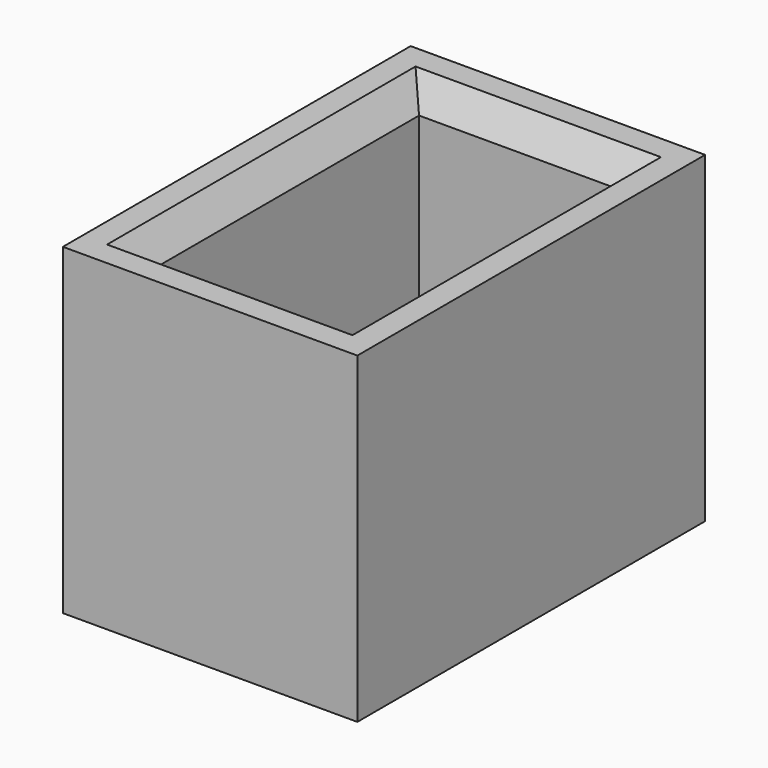
from build123d import *

# Parameters (mm, degrees)
F0_W         = 6
F0_H         = 10
F1_DEPTH     = 8
F2_T         = 1.2
F3_T1_DEPTH  = 6
F3_T3_DEPTH  = 10
F3_T9_DEPTH  = 8.2404819853
F3_T13_DEPTH = 12.2404819853
F3_T20_DEPTH = 8.2404819853
F3_T24_DEPTH = 12.2404819853
F3_T31_DEPTH = 12.2404819853
F3_T35_DEPTH = 8.2404819853
F3_T42_DEPTH = 8.2404819853
F3_T46_DEPTH = 12.2404819853


# Not quite as in the source:
# - a fillet or chamfer that OpenCascade refuses, or shapes differently, is made with other operations: its cross-section is extruded or revolved along the edge and cut away or added


with BuildPart() as f1:
    # F0 (on Top) → F1 (new body)
    with BuildSketch(Plane.XY):
        Rectangle(F0_W, F0_H)
    extrude(amount=F1_DEPTH)

    # F2
    f2_openings = [f1.faces().sort_by_distance(p)[0] for p in [
        (0, 0, 8),
    ]]
    offset(amount=F2_T, openings=f2_openings, kind=Kind.INTERSECTION)

    # F3: chamfer of 0.5 x 0.8660254038 on 4 edges, made by hand

    # F3_s2 → F3_t1 (cut)
    with BuildSketch(Plane.YZ.offset(-3)):
        Polygon((5, 7.1339745962), (5.5, 8), (5, 8), align=None)
        Polygon((-5, 7.1339745962), (-5.5, 8), (-5, 8), align=None)
    extrude(amount=F3_T1_DEPTH, mode=Mode.SUBTRACT)

    # F3_s4 → F3_t3 (cut)
    with BuildSketch(Plane.XZ.offset(-5)):
        Polygon((-3, 7.1339745962), (-3.5, 8), (-3, 8), align=None)
        Polygon((3, 7.1339745962), (3.5, 8), (3, 8), align=None)
    extrude(amount=F3_T3_DEPTH, mode=Mode.SUBTRACT)


with BuildPart() as f3_tool7:
    # F3_s8 → F3_t9 (new body)
    with BuildSketch(Plane.YZ.offset(5.2404819853)):
        Polygon((5, 7.1339745962), (5.5, 8), (5, 8), align=None)
    extrude(amount=-F3_T9_DEPTH)

    split(bisect_by=Plane.YZ.offset(3), keep=Keep.TOP)


with BuildPart() as f3_tool11:
    # F3_s12 → F3_t13 (new body)
    with BuildSketch(Plane.XZ.offset(5)):
        Polygon((3, 7.1339745962), (3.5, 8), (3, 8), align=None)
    extrude(amount=-F3_T13_DEPTH)

    split(bisect_by=Plane.XZ.offset(-5), keep=Keep.BOTTOM)


with BuildPart() as f3_tool7_1:
    add(f3_tool7.part)

    # F3_t15: intersect F3_tool11
    add(f3_tool11.part, mode=Mode.INTERSECT)


with BuildPart() as f1_1:
    add(f1.part)

    # F3_t5: cut F3_tool7
    add(f3_tool7_1.part, mode=Mode.SUBTRACT)


with BuildPart() as f3_tool18:
    # F3_s19 → F3_t20 (new body)
    with BuildSketch(Plane.YZ.offset(3)):
        Polygon((5, 7.1339745962), (5.5, 8), (5, 8), align=None)
    extrude(amount=-F3_T20_DEPTH)

    split(bisect_by=Plane.YZ.offset(-3), keep=Keep.BOTTOM)


with BuildPart() as f3_tool22:
    # F3_s23 → F3_t24 (new body)
    with BuildSketch(Plane.XZ.offset(-7.2404819853)):
        Polygon((-3, 7.1339745962), (-3.5, 8), (-3, 8), align=None)
    extrude(amount=F3_T24_DEPTH)

    split(bisect_by=Plane.XZ.offset(-5), keep=Keep.BOTTOM)


with BuildPart() as f3_tool18_1:
    add(f3_tool18.part)

    # F3_t26: intersect F3_tool22
    add(f3_tool22.part, mode=Mode.INTERSECT)


with BuildPart() as f1_2:
    add(f1_1.part)

    # F3_t16: cut F3_tool18
    add(f3_tool18_1.part, mode=Mode.SUBTRACT)


with BuildPart() as f3_tool29:
    # F3_s30 → F3_t31 (new body)
    with BuildSketch(Plane.XZ.offset(-5)):
        Polygon((-3, 7.1339745962), (-3.5, 8), (-3, 8), align=None)
    extrude(amount=F3_T31_DEPTH)

    split(bisect_by=Plane.XZ.offset(5), keep=Keep.TOP)


with BuildPart() as f3_tool33:
    # F3_s34 → F3_t35 (new body)
    with BuildSketch(Plane.YZ.offset(-5.2404819853)):
        Polygon((-5, 7.1339745962), (-5.5, 8), (-5, 8), align=None)
    extrude(amount=F3_T35_DEPTH)

    split(bisect_by=Plane.YZ.offset(-3), keep=Keep.BOTTOM)


with BuildPart() as f3_tool29_1:
    add(f3_tool29.part)

    # F3_t37: intersect F3_tool33
    add(f3_tool33.part, mode=Mode.INTERSECT)


with BuildPart() as f1_3:
    add(f1_2.part)

    # F3_t27: cut F3_tool29
    add(f3_tool29_1.part, mode=Mode.SUBTRACT)


with BuildPart() as f3_tool40:
    # F3_s41 → F3_t42 (new body)
    with BuildSketch(Plane.YZ.offset(-3)):
        Polygon((-5, 7.1339745962), (-5.5, 8), (-5, 8), align=None)
    extrude(amount=F3_T42_DEPTH)

    split(bisect_by=Plane.YZ.offset(3), keep=Keep.TOP)


with BuildPart() as f3_tool44:
    # F3_s45 → F3_t46 (new body)
    with BuildSketch(Plane.XZ.offset(7.2404819853)):
        Polygon((3, 7.1339745962), (3.5, 8), (3, 8), align=None)
    extrude(amount=-F3_T46_DEPTH)

    split(bisect_by=Plane.XZ.offset(5), keep=Keep.TOP)


with BuildPart() as f3_tool40_1:
    add(f3_tool40.part)

    # F3_t48: intersect F3_tool44
    add(f3_tool44.part, mode=Mode.INTERSECT)


with BuildPart() as f1_4:
    add(f1_3.part)

    # F3_t38: cut F3_tool40
    add(f3_tool40_1.part, mode=Mode.SUBTRACT)


solid = f1_4.part
